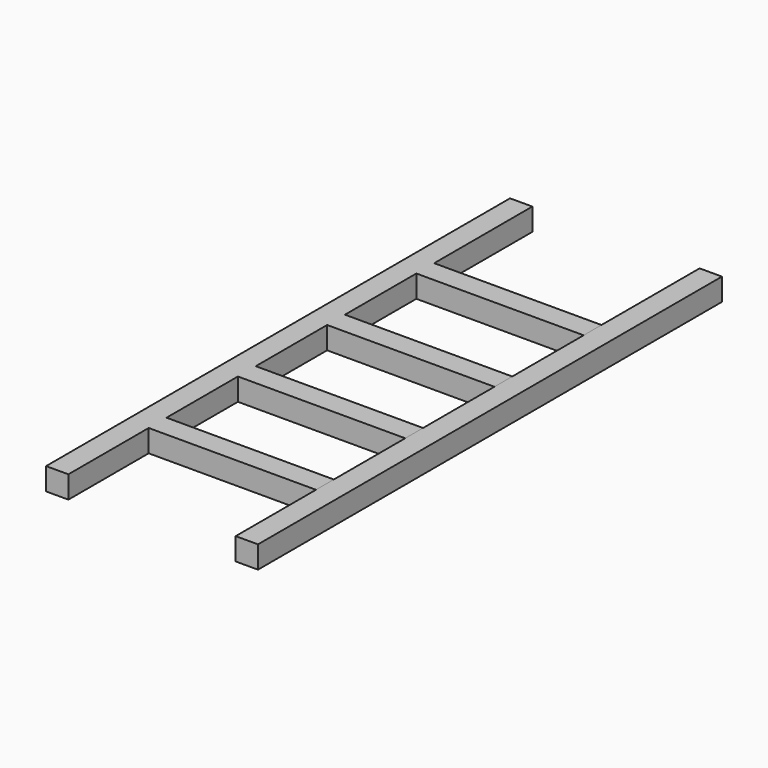
from build123d import *

# Parameters (mm, degrees)
F0_W     = 2
F0_H     = 2
F1_DEPTH = 52
F2_W     = 2
F2_H     = 2
F3_DEPTH = 15


with BuildPart() as f1:
    # F0 (on Front) → F1 (new body)
    with BuildSketch(Plane.XZ):
        with Locations((-29.2174071148, 15.274727294)):
            Rectangle(F0_W, F0_H)
    extrude(amount=F1_DEPTH)

    # F2 (on face) → F3 (join)
    with BuildSketch(Plane.YZ.offset(-28.2174071148)):
        with Locations((-42, 15.274727294)):
            Rectangle(F2_W, F2_H)
        with Locations((-32, 15.274727294)):
            Rectangle(F2_W, F2_H)
        with Locations((-22, 15.274727294)):
            Rectangle(F2_W, F2_H)
        with Locations((-12, 15.274727294)):
            Rectangle(F2_W, F2_H)
    extrude(amount=F3_DEPTH)


with BuildPart() as f1b:
    # F0 (on Front) → F1, piece 2 (new body)
    with BuildSketch(Plane.XZ):
        with Locations((-12.2174071148, 15.274727294)):
            Rectangle(F0_W, F0_H)
    extrude(amount=F1_DEPTH)


solid = Compound([f1.part, f1b.part])
